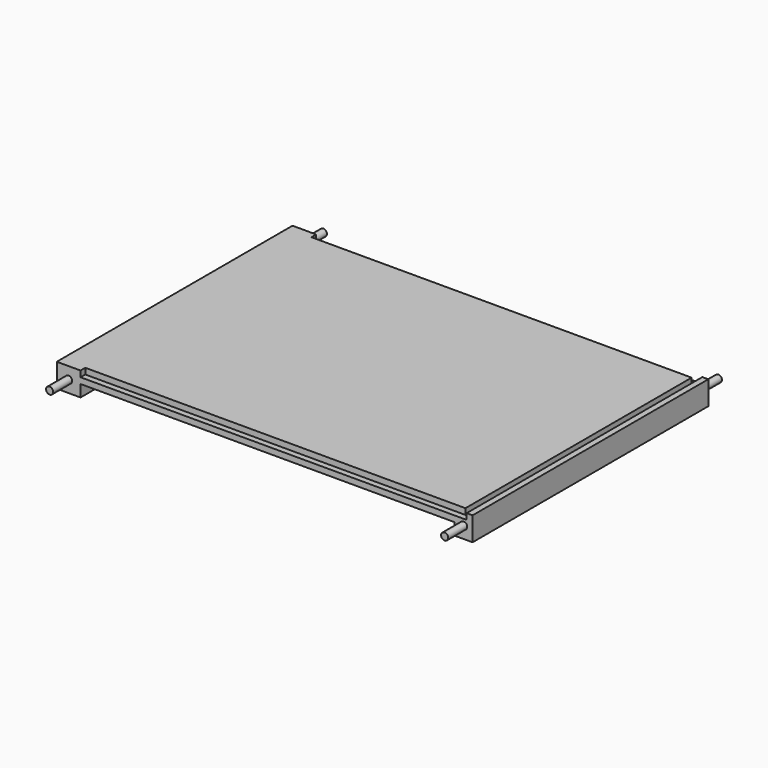
from build123d import *

# Parameters (mm, degrees)
F1_DEPTH = 496
F2_R     = 6
F3_DEPTH = 40
F5_W     = 650
F5_H     = 10
F6_DEPTH = 10
F7_W     = 10
F7_H     = 476
F8_DEPTH = 10


# Not quite as in the source:
# - a pattern or mirror of a feature is missing from the dataset's text; its kind, count and spacing are read off the source's solid


with BuildPart() as f1:
    # F0 (on Front) → F1 (new body)
    with BuildSketch(Plane.XZ):
        Polygon((374.2424272732, 0), (-325.7575727268, 0), (-325.7575727268, -40), (-285.7575727268, -40), (-285.7575727268, -20), (344.2424272732, -20), (344.2424272732, -40), (374.2424272732, -40), align=None)
    extrude(amount=F1_DEPTH)

    # F2 (on face) → F3 (join)
    with BuildSketch(Plane(origin=(0, 0, 0), x_dir=(-1, 0, 0), z_dir=(0, 1, 0))):
        with Locations((-359.2424272732, -20)):
            Circle(F2_R)
        with Locations((305.7575727268, -20)):
            Circle(F2_R)
    f3 = extrude(amount=F3_DEPTH)

    # F3_copies: F3 across plane
    add(f3.mirror(Plane(origin=(0, -248, 0), x_dir=(0, 0, -1), z_dir=(0, -1, 0))))

    # F5 (on face) → F6 (cut)
    with BuildSketch(Plane(origin=(0, 0, 0), x_dir=(-1, 0, 0), z_dir=(0, 1, 0))):
        with Locations((-39.2424272732, -5)):
            Rectangle(F5_W, F5_H)
    f6 = extrude(amount=-F6_DEPTH, mode=Mode.SUBTRACT)

    # F6_copies: F6 across plane
    add(f6.mirror(Plane(origin=(0, -248, 0), x_dir=(0, 0, -1), z_dir=(0, -1, 0))), mode=Mode.SUBTRACT)

    # F7 (on face) → F8 (cut)
    with BuildSketch(Plane.XY):
        with Locations((359.2424272732, -248)):
            Rectangle(F7_W, F7_H)
    extrude(amount=-F8_DEPTH, mode=Mode.SUBTRACT)


solid = f1.part
